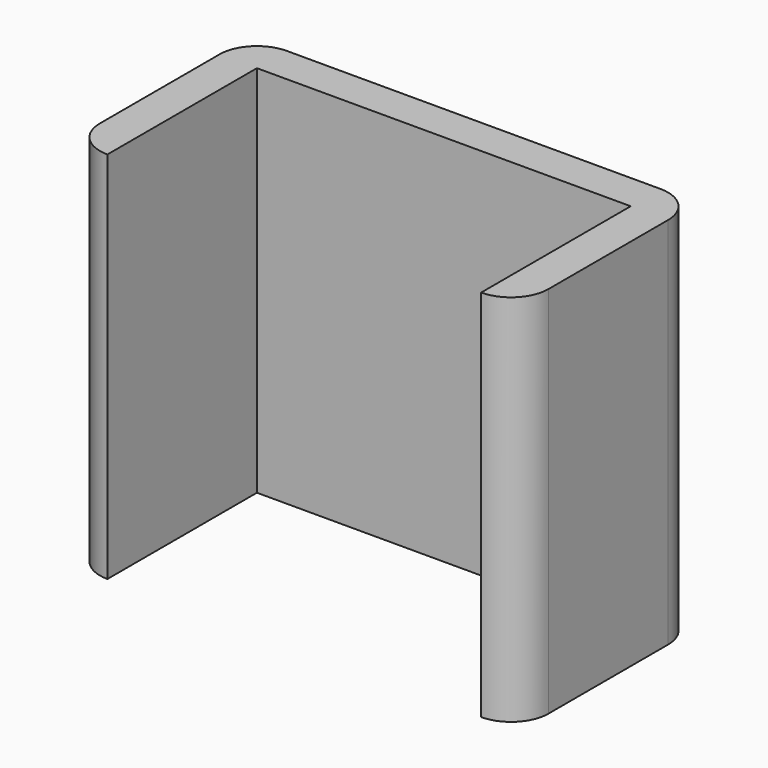
from build123d import *

# Parameters (mm, degrees)
F1_DEPTH      = 25
F1_DEPTH_BACK = 25
F2_R          = 4.99999


# Not quite as in the source:
# - a fillet or chamfer is up to 0.001 mm smaller than in the source, because OpenCascade refuses the exact size


with BuildPart() as f1:
    # F0 (on Top) → F1 (new body, two sides)
    with BuildSketch(Plane.XY) as f1_sk:
        Polygon((30, 15), (-30, 15), (-30, -15), (-25, -15), (-25, 10), (25, 10), (25, -15), (30, -15), align=None)
    extrude(amount=F1_DEPTH)
    extrude(f1_sk.sketch, amount=-F1_DEPTH_BACK)

    # F2 (radius 5 in the source; OpenCascade refuses exactly that, so slightly less here)
    f2_edges = [f1.edges().sort_by_distance(p)[0] for p in [
        (-30, 15, 0),
        (30, 15, 0),
        (30, -15, 0),
        (-30, -15, 0),
    ]]
    fillet(f2_edges, radius=F2_R)


solid = f1.part
